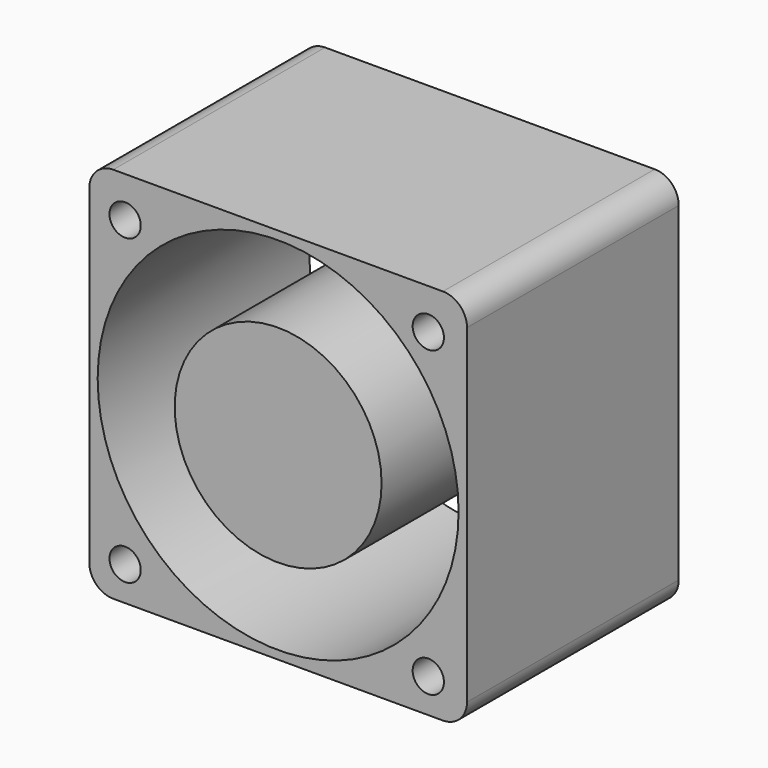
from build123d import *

# Parameters (mm, degrees)
F0_W     = 39.878
F0_H     = 39.878
F0_R     = 19.05
F2_DEPTH = 27.94
F0_R_2   = 10.922
F3_D     = 3.302
F4_R     = 2.54


# Not quite as in the source:
# - a feature names something its author has since deleted; it is built from what else it names


with BuildPart() as f2:
    # F0 (on Front) → F2 (new body)
    with BuildSketch(Plane.XZ):
        Rectangle(F0_W, F0_H)
        Circle(F0_R, mode=Mode.SUBTRACT)
    extrude(amount=F2_DEPTH)

    # F3 (through all)
    with Locations(Plane(origin=(0, 0, 0), x_dir=(1, 0, 0), z_dir=(0, 1, 0))):
        with Locations((15.8517888446, 16.3328610361), (15.8517888446, -15.6711389639), (-16.1522111554, 16.3328610361), (-16.1522111554, -15.6711389639)):
            Hole(F3_D / 2)

    # F4
    f4_edges = [f2.edges().sort_by_distance(p)[0] for p in [
        (19.939, -13.97, 19.939),
        (-19.939, -13.97, 19.939),
        (-19.939, -13.97, -19.939),
        (19.939, -13.97, -19.939),
    ]]
    fillet(f4_edges, radius=F4_R)


with BuildPart() as f2b:
    # F0 (on Front) → F2, piece 2 (new body)
    with BuildSketch(Plane.XZ):
        Circle(F0_R_2)
    extrude(amount=F2_DEPTH)


solid = Compound([f2.part, f2b.part])
